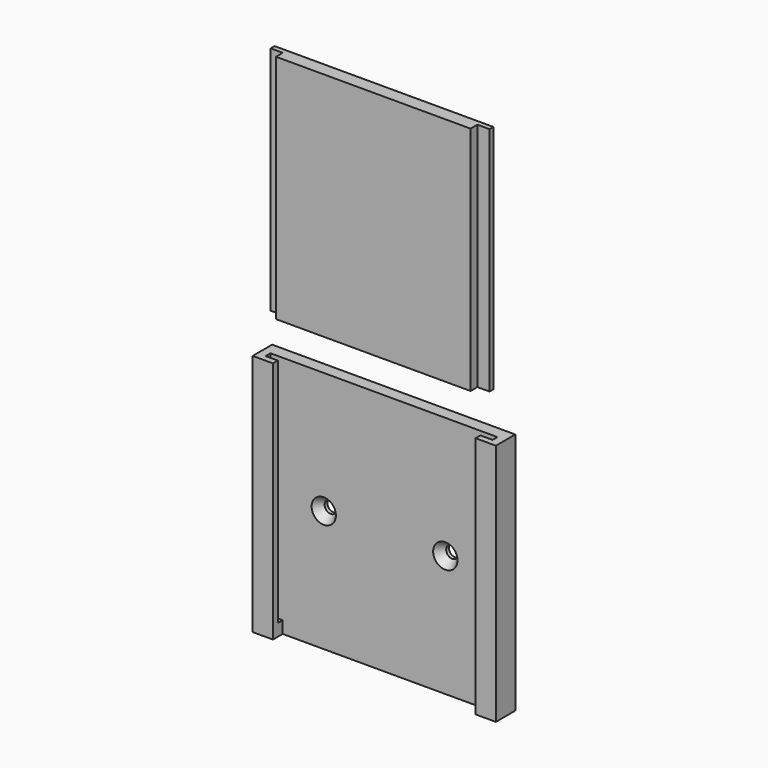
from build123d import *

# Parameters (mm, degrees)
F0_W           = 60
F0_H           = 60
F1_DEPTH       = 3
F2_W           = 2
F2_H           = 60
F3_DEPTH       = 3
F5_D           = 3
F5_CSINK_D     = 6
F5_CSINK_ANGLE = 70
F6_W           = 1.5
F6_H           = 3
F7_DEPTH       = 3
F8_W           = 1.5
F8_H           = 3
F9_DEPTH       = 3
F10_W          = 54
F10_H          = 57
F11_DEPTH      = 1.2
F12_W          = 48
F12_H          = 57
F13_DEPTH      = 2.1


# Not quite as in the source:
# - a feature names something its author has since deleted; it is built from what else it names


with BuildPart() as f1:
    # F0 (on Front) → F1 (new body)
    with BuildSketch(Plane.XZ):
        Rectangle(F0_W, F0_H)
    extrude(amount=F1_DEPTH)

    # F2 (on face) → F3 (join)
    with BuildSketch(Plane.XZ.offset(3)):
        with Locations((29, 0)):
            Rectangle(F2_W, F2_H)
        with Locations((-29, 0)):
            Rectangle(F2_W, F2_H)
    extrude(amount=F3_DEPTH)

    # F5 (through all)
    with Locations(Plane.XZ.offset(3)):
        with Locations((15.1334543969, 0), (-14.8665456031, 0)):
            CounterSinkHole(F5_D / 2, F5_CSINK_D / 2, counter_sink_angle=F5_CSINK_ANGLE)

    # F6 (on face) → F7 (join)
    with BuildSketch(Plane(origin=(28, 0, 0), x_dir=(0, -1, 0), z_dir=(-1, 0, 0))):
        Polygon((6, -30), (6, 30), (4.5, 30), (4.5, -27), (4.5, -30), align=None)
        with Locations((3.75, -28.5)):
            Rectangle(F6_W, F6_H)
    extrude(amount=F7_DEPTH)

    # F8 (on face) → F9 (join)
    with BuildSketch(Plane.YZ.offset(-28)):
        Polygon((-4.5, 30), (-6, 30), (-6, -30), (-4.5, -30), (-4.5, -27), align=None)
        with Locations((-3.75, -28.5)):
            Rectangle(F8_W, F8_H)
    extrude(amount=F9_DEPTH)


with BuildPart() as f11:
    # F10 (on face) → F11 (new body)
    with BuildSketch(Plane.XZ.offset(3)):
        with Locations((0, 68.5490723848)):
            Rectangle(F10_W, F10_H)
    extrude(amount=F11_DEPTH)

    # F12 (on face) → F13 (join)
    with BuildSketch(Plane.XZ.offset(4.2)):
        with Locations((0, 68.5490723848)):
            Rectangle(F12_W, F12_H)
    extrude(amount=F13_DEPTH)


solid = Compound([f1.part, f11.part])
